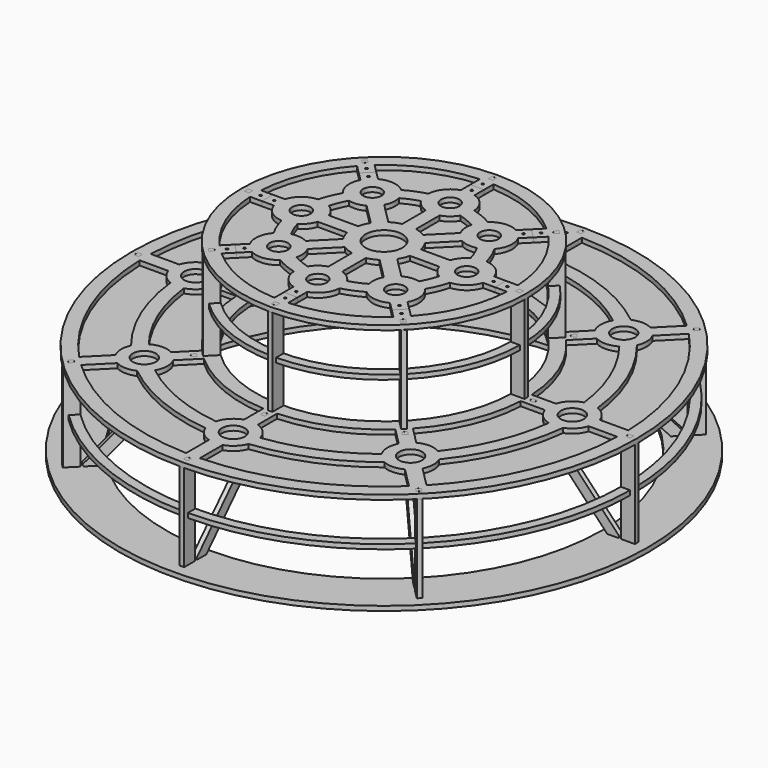
from build123d import *

# Parameters (mm, degrees)
F4_R      = 550
F4_R_2    = 25
F4_R_3    = 280
F5_DEPTH  = 10
F6_R      = 310
F6_R_2    = 2.5
F7_DEPTH  = 10
F8_R      = 575
F8_R_2    = 475
F9_DEPTH  = 10
F11_DEPTH = 5
F12_COUNT = 8
F13_R     = 520
F14_DEPTH = 10
F15_R     = 280
F16_DEPTH = 10
F17_COUNT = 8
F19_DEPTH = 1
F20_COUNT = 8
F6_R_3    = 20
F6_R_4    = 40
F21_DEPTH = 10
F23_DEPTH = 1
F24_COUNT = 4
F25_R     = 60
F26_DEPTH = 1


# Not quite as in the source:
# - the program builds the solid bodies; features that only make, move or delete a surface that nothing else refers to are left out


with BuildPart() as f5:
    # F4 (on Top) → F5 (new body)
    with BuildSketch(Plane.XY):
        Circle(F4_R)
        Polygon((-374.0594872477, -375.4737008101), (-371.3017708011, -378.2314172567), (-378.3728386129, -385.3024850685), (-381.1305550595, -382.5447686219), (-382.5447686219, -382.5447686219), (-382.5447686219, -381.1305550595), (-385.3024850685, -378.3728386129), (-378.2314172567, -371.3017708011), (-375.4737008101, -374.0594872477), (-374.0594872477, -374.0594872477), align=None, mode=Mode.SUBTRACT)
        with Locations((-289.9137802865, -289.9137802865)):
            Circle(F4_R_2, mode=Mode.SUBTRACT)
        with BuildLine():
            ThreePointArc((-46.8602222393, -427.4390243902), (-34.4319247471, -446.2552418033), (-15, -457.6969600708))
            Line((-15, -457.6969600708), (-15, -519.783608822))
            ThreePointArc((-15, -519.783608822), (-198.9953848298, -480.4173569059), (-356.9359128298, -378.1491162654))
            Line((-356.9359128298, -378.1491162654), (-313.0340224768, -334.2472259124))
            ThreePointArc((-313.0340224768, -334.2472259124), (-291.2030601412, -339.8971550971), (-269.1098517768, -335.3802136034))
            ThreePointArc((-269.1098517768, -335.3802136034), (-164.553875917, -397.2681989799), (-46.8602222393, -427.4390243902))
        make_face(mode=Mode.SUBTRACT)
        with BuildLine():
            Line((-15, -309.6368841078), (-15, -362.3030399292))
            ThreePointArc((-15, -362.3030399292), (-36.1104599854, -375.4162656782), (-48.3000733443, -397.0731707317))
            ThreePointArc((-48.3000733443, -397.0731707317), (-153.073372946, -369.5518130045), (-246.619822258, -314.9264410452))
            ThreePointArc((-246.619822258, -314.9264410452), (-239.9254361013, -290.9933383562), (-245.5803346606, -266.7935380962))
            Line((-245.5803346606, -266.7935380962), (-208.3397387403, -229.5529421759))
            ThreePointArc((-208.3397387403, -229.5529421759), (-118.6318640332, -286.4026550785), (-15, -309.6368841078))
        make_face(mode=Mode.SUBTRACT)
        with BuildLine():
            Line((-519.783608822, -15), (-457.6969600708, -15))
            ThreePointArc((-457.6969600708, -15), (-446.2552418033, -34.4319247471), (-427.4390243902, -46.8602222393))
            ThreePointArc((-427.4390243902, -46.8602222393), (-397.2681989799, -164.553875917), (-335.3802136034, -269.1098517768))
            ThreePointArc((-335.3802136034, -269.1098517768), (-339.8971550971, -291.2030601412), (-334.2472259124, -313.0340224768))
            Line((-334.2472259124, -313.0340224768), (-378.1491162654, -356.9359128298))
            ThreePointArc((-378.1491162654, -356.9359128298), (-480.4173569059, -198.9953848298), (-519.783608822, -15))
        make_face(mode=Mode.SUBTRACT)
        with BuildLine():
            ThreePointArc((-397.0731707317, -48.3000733443), (-375.4162656782, -36.1104599854), (-362.3030399292, -15))
            Line((-362.3030399292, -15), (-309.6368841078, -15))
            ThreePointArc((-309.6368841078, -15), (-286.4026550785, -118.6318640332), (-229.5529421759, -208.3397387403))
            Line((-229.5529421759, -208.3397387403), (-266.7935380962, -245.5803346606))
            ThreePointArc((-266.7935380962, -245.5803346606), (-290.9933383562, -239.9254361013), (-314.9264410452, -246.619822258))
            ThreePointArc((-314.9264410452, -246.619822258), (-369.5518130045, -153.073372946), (-397.0731707317, -48.3000733443))
        make_face(mode=Mode.SUBTRACT)
        Polygon((-236.8100610194, -229.8804145637), (-229.7389932075, -222.8093467519), (-226.9812767609, -225.5670631985), (-225.5670631985, -225.5670631985), (-225.5670631985, -226.9812767609), (-222.8093467519, -229.7389932075), (-229.8804145637, -236.8100610194), (-232.6381310104, -234.0523445727), (-234.0523445727, -234.0523445727), (-234.0523445727, -232.6381310104), align=None, mode=Mode.SUBTRACT)
        Polygon((-215.5968575838, -208.6672111282), (-208.5257897719, -201.5961433163), (-205.7680733253, -204.3538597629), (-204.3538597629, -204.3538597629), (-204.3538597629, -205.7680733253), (-201.5961433163, -208.5257897719), (-208.6672111282, -215.5968575838), (-211.4249275748, -212.8391411372), (-212.8391411372, -212.8391411372), (-212.8391411372, -211.4249275748), align=None, mode=Mode.SUBTRACT)
        Polygon((1, -530), (4.9, -530), (4.9, -540), (1, -540), (0, -541), (-1, -540), (-4.9, -540), (-4.9, -530), (-1, -530), (0, -529), align=None, mode=Mode.SUBTRACT)
        with BuildLine():
            ThreePointArc((356.9359128298, -378.1491162654), (198.9953848298, -480.4173569059), (15, -519.783608822))
            Line((15, -519.783608822), (15, -457.6969600708))
            ThreePointArc((15, -457.6969600708), (34.4319247471, -446.2552418033), (46.8602222393, -427.4390243902))
            ThreePointArc((46.8602222393, -427.4390243902), (164.553875917, -397.2681989799), (269.1098517768, -335.3802136034))
            ThreePointArc((269.1098517768, -335.3802136034), (291.2030601412, -339.8971550971), (313.0340224768, -334.2472259124))
            Line((313.0340224768, -334.2472259124), (356.9359128298, -378.1491162654))
        make_face(mode=Mode.SUBTRACT)
        with Locations((0, -410)):
            Circle(F4_R_2, mode=Mode.SUBTRACT)
        Polygon((-4.9, -330), (-4.9, -320), (-1, -320), (0, -319), (1, -320), (4.9, -320), (4.9, -330), (1, -330), (0, -331), (-1, -330), align=None, mode=Mode.SUBTRACT)
        Polygon((-4.9, -300), (-4.9, -290), (-1, -290), (0, -289), (1, -290), (4.9, -290), (4.9, -300), (1, -300), (0, -301), (-1, -300), align=None, mode=Mode.SUBTRACT)
        with BuildLine():
            ThreePointArc((246.619822258, -314.9264410452), (153.073372946, -369.5518130045), (48.3000733443, -397.0731707317))
            ThreePointArc((48.3000733443, -397.0731707317), (36.1104599854, -375.4162656782), (15, -362.3030399292))
            Line((15, -362.3030399292), (15, -309.6368841078))
            ThreePointArc((15, -309.6368841078), (118.6318640332, -286.4026550785), (208.3397387403, -229.5529421759))
            Line((208.3397387403, -229.5529421759), (245.5803346606, -266.7935380962))
            ThreePointArc((245.5803346606, -266.7935380962), (239.9254361013, -290.9933383562), (246.619822258, -314.9264410452))
        make_face(mode=Mode.SUBTRACT)
        Polygon((375.4737008101, -374.0594872477), (378.2314172567, -371.3017708011), (385.3024850685, -378.3728386129), (382.5447686219, -381.1305550595), (382.5447686219, -382.5447686219), (381.1305550595, -382.5447686219), (378.3728386129, -385.3024850685), (371.3017708011, -378.2314172567), (374.0594872477, -375.4737008101), (374.0594872477, -374.0594872477), align=None, mode=Mode.SUBTRACT)
        with Locations((289.9137802865, -289.9137802865)):
            Circle(F4_R_2, mode=Mode.SUBTRACT)
        Polygon((229.8804145637, -236.8100610194), (222.8093467519, -229.7389932075), (225.5670631985, -226.9812767609), (225.5670631985, -225.5670631985), (226.9812767609, -225.5670631985), (229.7389932075, -222.8093467519), (236.8100610194, -229.8804145637), (234.0523445727, -232.6381310104), (234.0523445727, -234.0523445727), (232.6381310104, -234.0523445727), align=None, mode=Mode.SUBTRACT)
        Polygon((208.6672111282, -215.5968575838), (201.5961433163, -208.5257897719), (204.3538597629, -205.7680733253), (204.3538597629, -204.3538597629), (205.7680733253, -204.3538597629), (208.5257897719, -201.5961433163), (215.5968575838, -208.6672111282), (212.8391411372, -211.4249275748), (212.8391411372, -212.8391411372), (211.4249275748, -212.8391411372), align=None, mode=Mode.SUBTRACT)
        with BuildLine():
            Line((378.1491162654, -356.9359128298), (334.2472259124, -313.0340224768))
            ThreePointArc((334.2472259124, -313.0340224768), (339.8971550971, -291.2030601412), (335.3802136034, -269.1098517768))
            ThreePointArc((335.3802136034, -269.1098517768), (397.2681989799, -164.553875917), (427.4390243902, -46.8602222393))
            ThreePointArc((427.4390243902, -46.8602222393), (446.2552418033, -34.4319247471), (457.6969600708, -15))
            Line((457.6969600708, -15), (519.783608822, -15))
            ThreePointArc((519.783608822, -15), (480.4173569059, -198.9953848298), (378.1491162654, -356.9359128298))
        make_face(mode=Mode.SUBTRACT)
        with BuildLine():
            ThreePointArc((314.9264410452, -246.619822258), (290.9933383562, -239.9254361013), (266.7935380962, -245.5803346606))
            Line((266.7935380962, -245.5803346606), (229.5529421759, -208.3397387403))
            ThreePointArc((229.5529421759, -208.3397387403), (286.4026550785, -118.6318640332), (309.6368841078, -15))
            Line((309.6368841078, -15), (362.3030399292, -15))
            ThreePointArc((362.3030399292, -15), (375.4162656782, -36.1104599854), (397.0731707317, -48.3000733443))
            ThreePointArc((397.0731707317, -48.3000733443), (369.5518130045, -153.073372946), (314.9264410452, -246.619822258))
        make_face(mode=Mode.SUBTRACT)
        Polygon((-530, -1), (-530, -4.9), (-540, -4.9), (-540, -1), (-541, 0), (-540, 1), (-540, 4.9), (-530, 4.9), (-530, 1), (-529, 0), align=None, mode=Mode.SUBTRACT)
        with Locations((-410, 0)):
            Circle(F4_R_2, mode=Mode.SUBTRACT)
        Polygon((-330, 4.9), (-320, 4.9), (-320, 1), (-319, 0), (-320, -1), (-320, -4.9), (-330, -4.9), (-330, -1), (-331, 0), (-330, 1), align=None, mode=Mode.SUBTRACT)
        Polygon((-300, 4.9), (-290, 4.9), (-290, 1), (-289, 0), (-290, -1), (-290, -4.9), (-300, -4.9), (-300, -1), (-301, 0), (-300, 1), align=None, mode=Mode.SUBTRACT)
        with BuildLine():
            ThreePointArc((-314.9264410452, 246.619822258), (-290.9933383562, 239.9254361013), (-266.7935380962, 245.5803346606))
            Line((-266.7935380962, 245.5803346606), (-229.5529421759, 208.3397387403))
            ThreePointArc((-229.5529421759, 208.3397387403), (-286.4026550785, 118.6318640332), (-309.6368841078, 15))
            Line((-309.6368841078, 15), (-362.3030399292, 15))
            ThreePointArc((-362.3030399292, 15), (-375.4162656782, 36.1104599854), (-397.0731707317, 48.3000733443))
            ThreePointArc((-397.0731707317, 48.3000733443), (-369.5518130045, 153.073372946), (-314.9264410452, 246.619822258))
        make_face(mode=Mode.SUBTRACT)
        with BuildLine():
            Line((-378.1491162654, 356.9359128298), (-334.2472259124, 313.0340224768))
            ThreePointArc((-334.2472259124, 313.0340224768), (-339.8971550971, 291.2030601412), (-335.3802136034, 269.1098517768))
            ThreePointArc((-335.3802136034, 269.1098517768), (-397.2681989799, 164.553875917), (-427.4390243902, 46.8602222393))
            ThreePointArc((-427.4390243902, 46.8602222393), (-446.2552418033, 34.4319247471), (-457.6969600708, 15))
            Line((-457.6969600708, 15), (-519.783608822, 15))
            ThreePointArc((-519.783608822, 15), (-480.4173569059, 198.9953848298), (-378.1491162654, 356.9359128298))
        make_face(mode=Mode.SUBTRACT)
        Polygon((-208.6672111282, 215.5968575838), (-201.5961433163, 208.5257897719), (-204.3538597629, 205.7680733253), (-204.3538597629, 204.3538597629), (-205.7680733253, 204.3538597629), (-208.5257897719, 201.5961433163), (-215.5968575838, 208.6672111282), (-212.8391411372, 211.4249275748), (-212.8391411372, 212.8391411372), (-211.4249275748, 212.8391411372), align=None, mode=Mode.SUBTRACT)
        Polygon((-229.8804145637, 236.8100610194), (-222.8093467519, 229.7389932075), (-225.5670631985, 226.9812767609), (-225.5670631985, 225.5670631985), (-226.9812767609, 225.5670631985), (-229.7389932075, 222.8093467519), (-236.8100610194, 229.8804145637), (-234.0523445727, 232.6381310104), (-234.0523445727, 234.0523445727), (-232.6381310104, 234.0523445727), align=None, mode=Mode.SUBTRACT)
        with Locations((-289.9137802865, 289.9137802865)):
            Circle(F4_R_2, mode=Mode.SUBTRACT)
        Polygon((-375.4737008101, 374.0594872477), (-378.2314172567, 371.3017708011), (-385.3024850685, 378.3728386129), (-382.5447686219, 381.1305550595), (-382.5447686219, 382.5447686219), (-381.1305550595, 382.5447686219), (-378.3728386129, 385.3024850685), (-371.3017708011, 378.2314172567), (-374.0594872477, 375.4737008101), (-374.0594872477, 374.0594872477), align=None, mode=Mode.SUBTRACT)
        with BuildLine():
            ThreePointArc((-48.3000733443, 397.0731707317), (-36.1104599854, 375.4162656782), (-15, 362.3030399292))
            Line((-15, 362.3030399292), (-15, 309.6368841078))
            ThreePointArc((-15, 309.6368841078), (-118.6318640332, 286.4026550785), (-208.3397387403, 229.5529421759))
            Line((-208.3397387403, 229.5529421759), (-245.5803346606, 266.7935380962))
            ThreePointArc((-245.5803346606, 266.7935380962), (-239.9254361013, 290.9933383562), (-246.619822258, 314.9264410452))
            ThreePointArc((-246.619822258, 314.9264410452), (-153.073372946, 369.5518130045), (-48.3000733443, 397.0731707317))
        make_face(mode=Mode.SUBTRACT)
        with BuildLine():
            Line((-15, 519.783608822), (-15, 457.6969600708))
            ThreePointArc((-15, 457.6969600708), (-34.4319247471, 446.2552418033), (-46.8602222393, 427.4390243902))
            ThreePointArc((-46.8602222393, 427.4390243902), (-164.553875917, 397.2681989799), (-269.1098517768, 335.3802136034))
            ThreePointArc((-269.1098517768, 335.3802136034), (-291.2030601412, 339.8971550971), (-313.0340224768, 334.2472259124))
            Line((-313.0340224768, 334.2472259124), (-356.9359128298, 378.1491162654))
            ThreePointArc((-356.9359128298, 378.1491162654), (-198.9953848298, 480.4173569059), (-15, 519.783608822))
        make_face(mode=Mode.SUBTRACT)
        Circle(F4_R_3, mode=Mode.SUBTRACT)
        Polygon((215.5968575838, 208.6672111282), (208.5257897719, 201.5961433163), (205.7680733253, 204.3538597629), (204.3538597629, 204.3538597629), (204.3538597629, 205.7680733253), (201.5961433163, 208.5257897719), (208.6672111282, 215.5968575838), (211.4249275748, 212.8391411372), (212.8391411372, 212.8391411372), (212.8391411372, 211.4249275748), align=None, mode=Mode.SUBTRACT)
        Polygon((236.8100610194, 229.8804145637), (229.7389932075, 222.8093467519), (226.9812767609, 225.5670631985), (225.5670631985, 225.5670631985), (225.5670631985, 226.9812767609), (222.8093467519, 229.7389932075), (229.8804145637, 236.8100610194), (232.6381310104, 234.0523445727), (234.0523445727, 234.0523445727), (234.0523445727, 232.6381310104), align=None, mode=Mode.SUBTRACT)
        Polygon((300, -4.9), (290, -4.9), (290, -1), (289, 0), (290, 1), (290, 4.9), (300, 4.9), (300, 1), (301, 0), (300, -1), align=None, mode=Mode.SUBTRACT)
        Polygon((330, -4.9), (320, -4.9), (320, -1), (319, 0), (320, 1), (320, 4.9), (330, 4.9), (330, 1), (331, 0), (330, -1), align=None, mode=Mode.SUBTRACT)
        with Locations((410, 0)):
            Circle(F4_R_2, mode=Mode.SUBTRACT)
        with BuildLine():
            ThreePointArc((397.0731707317, 48.3000733443), (375.4162656782, 36.1104599854), (362.3030399292, 15))
            Line((362.3030399292, 15), (309.6368841078, 15))
            ThreePointArc((309.6368841078, 15), (286.4026550785, 118.6318640332), (229.5529421759, 208.3397387403))
            Line((229.5529421759, 208.3397387403), (266.7935380962, 245.5803346606))
            ThreePointArc((266.7935380962, 245.5803346606), (290.9933383562, 239.9254361013), (314.9264410452, 246.619822258))
            ThreePointArc((314.9264410452, 246.619822258), (369.5518130045, 153.073372946), (397.0731707317, 48.3000733443))
        make_face(mode=Mode.SUBTRACT)
        Polygon((530, 1), (530, 4.9), (540, 4.9), (540, 1), (541, 0), (540, -1), (540, -4.9), (530, -4.9), (530, -1), (529, 0), align=None, mode=Mode.SUBTRACT)
        with BuildLine():
            Line((519.783608822, 15), (457.6969600708, 15))
            ThreePointArc((457.6969600708, 15), (446.2552418033, 34.4319247471), (427.4390243902, 46.8602222393))
            ThreePointArc((427.4390243902, 46.8602222393), (397.2681989799, 164.553875917), (335.3802136034, 269.1098517768))
            ThreePointArc((335.3802136034, 269.1098517768), (339.8971550971, 291.2030601412), (334.2472259124, 313.0340224768))
            Line((334.2472259124, 313.0340224768), (378.1491162654, 356.9359128298))
            ThreePointArc((378.1491162654, 356.9359128298), (480.4173569059, 198.9953848298), (519.783608822, 15))
        make_face(mode=Mode.SUBTRACT)
        Polygon((4.9, 300), (4.9, 290), (1, 290), (0, 289), (-1, 290), (-4.9, 290), (-4.9, 300), (-1, 300), (0, 301), (1, 300), align=None, mode=Mode.SUBTRACT)
        Polygon((4.9, 330), (4.9, 320), (1, 320), (0, 319), (-1, 320), (-4.9, 320), (-4.9, 330), (-1, 330), (0, 331), (1, 330), align=None, mode=Mode.SUBTRACT)
        with BuildLine():
            ThreePointArc((246.619822258, 314.9264410452), (239.9254361013, 290.9933383562), (245.5803346606, 266.7935380962))
            Line((245.5803346606, 266.7935380962), (208.3397387403, 229.5529421759))
            ThreePointArc((208.3397387403, 229.5529421759), (118.6318640332, 286.4026550785), (15, 309.6368841078))
            Line((15, 309.6368841078), (15, 362.3030399292))
            ThreePointArc((15, 362.3030399292), (36.1104599854, 375.4162656782), (48.3000733443, 397.0731707317))
            ThreePointArc((48.3000733443, 397.0731707317), (153.073372946, 369.5518130045), (246.619822258, 314.9264410452))
        make_face(mode=Mode.SUBTRACT)
        with Locations((0, 410)):
            Circle(F4_R_2, mode=Mode.SUBTRACT)
        Polygon((4.9, 540), (4.9, 530), (1, 530), (0, 529), (-1, 530), (-4.9, 530), (-4.9, 540), (-1, 540), (0, 541), (1, 540), align=None, mode=Mode.SUBTRACT)
        with BuildLine():
            Line((356.9359128298, 378.1491162654), (313.0340224768, 334.2472259124))
            ThreePointArc((313.0340224768, 334.2472259124), (291.2030601412, 339.8971550971), (269.1098517768, 335.3802136034))
            ThreePointArc((269.1098517768, 335.3802136034), (164.553875917, 397.2681989799), (46.8602222393, 427.4390243902))
            ThreePointArc((46.8602222393, 427.4390243902), (34.4319247471, 446.2552418033), (15, 457.6969600708))
            Line((15, 457.6969600708), (15, 519.783608822))
            ThreePointArc((15, 519.783608822), (198.9953848298, 480.4173569059), (356.9359128298, 378.1491162654))
        make_face(mode=Mode.SUBTRACT)
        with Locations((289.9137802865, 289.9137802865)):
            Circle(F4_R_2, mode=Mode.SUBTRACT)
        Polygon((374.0594872477, 375.4737008101), (371.3017708011, 378.2314172567), (378.3728386129, 385.3024850685), (381.1305550595, 382.5447686219), (382.5447686219, 382.5447686219), (382.5447686219, 381.1305550595), (385.3024850685, 378.3728386129), (378.2314172567, 371.3017708011), (375.4737008101, 374.0594872477), (374.0594872477, 374.0594872477), align=None, mode=Mode.SUBTRACT)
    extrude(amount=F5_DEPTH)


with BuildPart() as f7:
    # F6 (on offset) → F7 (new body)
    with BuildSketch(Plane.XY.offset(200)):
        Circle(F6_R)
        Polygon((-204.3538597629, -204.3538597629), (-204.3538597629, -205.7680733253), (-201.5961433163, -208.5257897719), (-208.6672111282, -215.5968575838), (-211.4249275748, -212.8391411372), (-212.8391411372, -212.8391411372), (-212.8391411372, -211.4249275748), (-215.5968575838, -208.6672111282), (-208.5257897719, -201.5961433163), (-205.7680733253, -204.3538597629), align=None, mode=Mode.SUBTRACT)
        with Locations((-189.9624285775, -189.9624285775)):
            Circle(F6_R_2, mode=Mode.SUBTRACT)
        Polygon((0, -289), (1, -290), (4.9, -290), (4.9, -300), (1, -300), (0, -301), (-1, -300), (-4.9, -300), (-4.9, -290), (-1, -290), align=None, mode=Mode.SUBTRACT)
        with Locations((0, -268.6474428356)):
            Circle(F6_R_2, mode=Mode.SUBTRACT)
        Polygon((204.3538597629, -204.3538597629), (205.7680733253, -204.3538597629), (208.5257897719, -201.5961433163), (215.5968575838, -208.6672111282), (212.8391411372, -211.4249275748), (212.8391411372, -212.8391411372), (211.4249275748, -212.8391411372), (208.6672111282, -215.5968575838), (201.5961433163, -208.5257897719), (204.3538597629, -205.7680733253), align=None, mode=Mode.SUBTRACT)
        with Locations((189.9624285775, -189.9624285775)):
            Circle(F6_R_2, mode=Mode.SUBTRACT)
        Polygon((-289, 0), (-290, -1), (-290, -4.9), (-300, -4.9), (-300, -1), (-301, 0), (-300, 1), (-300, 4.9), (-290, 4.9), (-290, 1), align=None, mode=Mode.SUBTRACT)
        with Locations((-268.6474428356, 0)):
            Circle(F6_R_2, mode=Mode.SUBTRACT)
        with Locations((-189.9624285775, 189.9624285775)):
            Circle(F6_R_2, mode=Mode.SUBTRACT)
        Polygon((-204.3538597629, 204.3538597629), (-205.7680733253, 204.3538597629), (-208.5257897719, 201.5961433163), (-215.5968575838, 208.6672111282), (-212.8391411372, 211.4249275748), (-212.8391411372, 212.8391411372), (-211.4249275748, 212.8391411372), (-208.6672111282, 215.5968575838), (-201.5961433163, 208.5257897719), (-204.3538597629, 205.7680733253), align=None, mode=Mode.SUBTRACT)
        with BuildLine():
            Line((15, -279.5979256003), (15, -253.6474428356))
            Line((15, -253.6474428356), (-15, -253.6474428356))
            Line((-15, -253.6474428356), (-15, -279.5979256003))
            ThreePointArc((-15, -279.5979256003), (-107.1513610622, -258.6862691032), (-187.0989874799, -208.3121909155))
            Line((-187.0989874799, -208.3121909155), (-168.7492251419, -189.9624285775))
            Line((-168.7492251419, -189.9624285775), (-189.9624285775, -168.7492251419))
            Line((-189.9624285775, -168.7492251419), (-208.3121909155, -187.0989874799))
            ThreePointArc((-208.3121909155, -187.0989874799), (-258.6862691032, -107.1513610622), (-279.5979256003, -15))
            Line((-279.5979256003, -15), (-253.6474428356, -15))
            Line((-253.6474428356, -15), (-253.6474428356, 15))
            Line((-253.6474428356, 15), (-279.5979256003, 15))
            ThreePointArc((-279.5979256003, 15), (-258.6862691032, 107.1513610622), (-208.3121909155, 187.0989874799))
            Line((-208.3121909155, 187.0989874799), (-189.9624285775, 168.7492251419))
            Line((-189.9624285775, 168.7492251419), (-168.7492251419, 189.9624285775))
            Line((-168.7492251419, 189.9624285775), (-187.0989874799, 208.3121909155))
            ThreePointArc((-187.0989874799, 208.3121909155), (-107.1513610622, 258.6862691032), (-15, 279.5979256003))
            Line((-15, 279.5979256003), (-15, 253.6474428356))
            Line((-15, 253.6474428356), (15, 253.6474428356))
            Line((15, 253.6474428356), (15, 279.5979256003))
            ThreePointArc((15, 279.5979256003), (107.1513610622, 258.6862691032), (187.0989874799, 208.3121909155))
            Line((187.0989874799, 208.3121909155), (168.7492251419, 189.9624285775))
            Line((168.7492251419, 189.9624285775), (189.9624285775, 168.7492251419))
            Line((189.9624285775, 168.7492251419), (208.3121909155, 187.0989874799))
            ThreePointArc((208.3121909155, 187.0989874799), (258.6862691032, 107.1513610622), (279.5979256003, 15))
            Line((279.5979256003, 15), (253.6474428356, 15))
            Line((253.6474428356, 15), (253.6474428356, -15))
            Line((253.6474428356, -15), (279.5979256003, -15))
            ThreePointArc((279.5979256003, -15), (258.6862691032, -107.1513610622), (208.3121909155, -187.0989874799))
            Line((208.3121909155, -187.0989874799), (189.9624285775, -168.7492251419))
            Line((189.9624285775, -168.7492251419), (168.7492251419, -189.9624285775))
            Line((168.7492251419, -189.9624285775), (187.0989874799, -208.3121909155))
            ThreePointArc((187.0989874799, -208.3121909155), (107.1513610622, -258.6862691032), (15, -279.5979256003))
        make_face(mode=Mode.SUBTRACT)
        with Locations((268.6474428356, 0)):
            Circle(F6_R_2, mode=Mode.SUBTRACT)
        Polygon((289, 0), (290, 1), (290, 4.9), (300, 4.9), (300, 1), (301, 0), (300, -1), (300, -4.9), (290, -4.9), (290, -1), align=None, mode=Mode.SUBTRACT)
        with Locations((0, 268.6474428356)):
            Circle(F6_R_2, mode=Mode.SUBTRACT)
        Polygon((-1, 290), (-4.9, 290), (-4.9, 300), (-1, 300), (0, 301), (1, 300), (4.9, 300), (4.9, 290), (1, 290), (0, 289), align=None, mode=Mode.SUBTRACT)
        with Locations((189.9624285775, 189.9624285775)):
            Circle(F6_R_2, mode=Mode.SUBTRACT)
        Polygon((204.3538597629, 204.3538597629), (204.3538597629, 205.7680733253), (201.5961433163, 208.5257897719), (208.6672111282, 215.5968575838), (211.4249275748, 212.8391411372), (212.8391411372, 212.8391411372), (212.8391411372, 211.4249275748), (215.5968575838, 208.6672111282), (208.5257897719, 201.5961433163), (205.7680733253, 204.3538597629), align=None, mode=Mode.SUBTRACT)
    extrude(amount=F7_DEPTH)


with BuildPart() as f9:
    # F8 (on offset) → F9 (new body)
    with BuildSketch(Plane.XY.offset(-200)):
        Circle(F8_R)
        Polygon((-374.0594872477, -375.4737008101), (-371.3017708011, -378.2314172567), (-378.3728386129, -385.3024850685), (-381.1305550595, -382.5447686219), (-382.5447686219, -382.5447686219), (-382.5447686219, -381.1305550595), (-385.3024850685, -378.3728386129), (-378.2314172567, -371.3017708011), (-375.4737008101, -374.0594872477), (-374.0594872477, -374.0594872477), align=None, mode=Mode.SUBTRACT)
        Polygon((-364.089281633, -357.1596351773), (-357.0182138211, -350.0885673655), (-354.2604973745, -352.8462838121), (-352.8462838121, -352.8462838121), (-352.8462838121, -354.2604973745), (-350.0885673655, -357.0182138211), (-357.1596351773, -364.089281633), (-359.917351624, -361.3315651863), (-361.3315651863, -361.3315651863), (-361.3315651863, -359.917351624), align=None, mode=Mode.SUBTRACT)
        Polygon((1, -530), (4.9, -530), (4.9, -540), (1, -540), (0, -541), (-1, -540), (-4.9, -540), (-4.9, -530), (-1, -530), (0, -529), align=None, mode=Mode.SUBTRACT)
        Polygon((-4.9, -510), (-4.9, -500), (-1, -500), (0, -499), (1, -500), (4.9, -500), (4.9, -510), (1, -510), (0, -511), (-1, -510), align=None, mode=Mode.SUBTRACT)
        Polygon((375.4737008101, -374.0594872477), (378.2314172567, -371.3017708011), (385.3024850685, -378.3728386129), (382.5447686219, -381.1305550595), (382.5447686219, -382.5447686219), (381.1305550595, -382.5447686219), (378.3728386129, -385.3024850685), (371.3017708011, -378.2314172567), (374.0594872477, -375.4737008101), (374.0594872477, -374.0594872477), align=None, mode=Mode.SUBTRACT)
        Polygon((357.1596351773, -364.089281633), (350.0885673655, -357.0182138211), (352.8462838121, -354.2604973745), (352.8462838121, -352.8462838121), (354.2604973745, -352.8462838121), (357.0182138211, -350.0885673655), (364.089281633, -357.1596351773), (361.3315651863, -359.917351624), (361.3315651863, -361.3315651863), (359.917351624, -361.3315651863), align=None, mode=Mode.SUBTRACT)
        Polygon((-530, -1), (-530, -4.9), (-540, -4.9), (-540, -1), (-541, 0), (-540, 1), (-540, 4.9), (-530, 4.9), (-530, 1), (-529, 0), align=None, mode=Mode.SUBTRACT)
        Polygon((-510, 4.9), (-500, 4.9), (-500, 1), (-499, 0), (-500, -1), (-500, -4.9), (-510, -4.9), (-510, -1), (-511, 0), (-510, 1), align=None, mode=Mode.SUBTRACT)
        Polygon((-357.1596351773, 364.089281633), (-350.0885673655, 357.0182138211), (-352.8462838121, 354.2604973745), (-352.8462838121, 352.8462838121), (-354.2604973745, 352.8462838121), (-357.0182138211, 350.0885673655), (-364.089281633, 357.1596351773), (-361.3315651863, 359.917351624), (-361.3315651863, 361.3315651863), (-359.917351624, 361.3315651863), align=None, mode=Mode.SUBTRACT)
        Polygon((-375.4737008101, 374.0594872477), (-378.2314172567, 371.3017708011), (-385.3024850685, 378.3728386129), (-382.5447686219, 381.1305550595), (-382.5447686219, 382.5447686219), (-381.1305550595, 382.5447686219), (-378.3728386129, 385.3024850685), (-371.3017708011, 378.2314172567), (-374.0594872477, 375.4737008101), (-374.0594872477, 374.0594872477), align=None, mode=Mode.SUBTRACT)
        Circle(F8_R_2, mode=Mode.SUBTRACT)
        Polygon((510, -4.9), (500, -4.9), (500, -1), (499, 0), (500, 1), (500, 4.9), (510, 4.9), (510, 1), (511, 0), (510, -1), align=None, mode=Mode.SUBTRACT)
        Polygon((530, 1), (530, 4.9), (540, 4.9), (540, 1), (541, 0), (540, -1), (540, -4.9), (530, -4.9), (530, -1), (529, 0), align=None, mode=Mode.SUBTRACT)
        Polygon((4.9, 510), (4.9, 500), (1, 500), (0, 499), (-1, 500), (-4.9, 500), (-4.9, 510), (-1, 510), (0, 511), (1, 510), align=None, mode=Mode.SUBTRACT)
        Polygon((4.9, 540), (4.9, 530), (1, 530), (0, 529), (-1, 530), (-4.9, 530), (-4.9, 540), (-1, 540), (0, 541), (1, 540), align=None, mode=Mode.SUBTRACT)
        Polygon((364.089281633, 357.1596351773), (357.0182138211, 350.0885673655), (354.2604973745, 352.8462838121), (352.8462838121, 352.8462838121), (352.8462838121, 354.2604973745), (350.0885673655, 357.0182138211), (357.1596351773, 364.089281633), (359.917351624, 361.3315651863), (361.3315651863, 361.3315651863), (361.3315651863, 359.917351624), align=None, mode=Mode.SUBTRACT)
        Polygon((374.0594872477, 375.4737008101), (371.3017708011, 378.2314172567), (378.3728386129, 385.3024850685), (381.1305550595, 382.5447686219), (382.5447686219, 382.5447686219), (382.5447686219, 381.1305550595), (385.3024850685, 378.3728386129), (378.2314172567, 371.3017708011), (375.4737008101, 374.0594872477), (374.0594872477, 374.0594872477), align=None, mode=Mode.SUBTRACT)
    extrude(amount=F9_DEPTH)


with BuildPart() as f11:
    # F10 (on Right) → F11 (new body, symmetric)
    with BuildSketch(Plane.YZ):
        Polygon((550, 0), (540, 0), (540, 10), (530, 10), (530, 0), (520, 0), (520, -90.1), (530, -90.1), (530, -99.9), (520, -99.9), (520, -190), (530, -190), (530, -200), (540, -200), (540, -190), (550, -190), align=None)
    extrude(amount=F11_DEPTH, both=True)


with BuildPart() as f11b:
    # F10 (on Right) → F11, piece 2 (new body, symmetric)
    with BuildSketch(Plane.YZ):
        Polygon((290, 10), (290, 0), (300, 0), (300, 10), (310, 10), (310, 200), (300, 200), (300, 210), (290, 210), (290, 200), (280, 200), (280, 109.9), (290, 109.9), (290, 100.1), (280, 100.1), (280, 10), align=None)
    extrude(amount=F11_DEPTH, both=True)


with BuildPart() as f11c:
    # F10 (on Right) → F11, piece 3 (new body, symmetric)
    with BuildSketch(Plane.YZ):
        with BuildLine():
            Line((510, -190), (513.0253940016, -190))
            ThreePointArc((513.0253940016, -190), (515.7812697092, -188.1853898449), (515.2032520533, -184.9367660563))
            Line((515.2032520533, -184.9367660563), (340, 0))
            Line((340, 0), (330, 0))
            Line((330, 0), (330, 10))
            Line((330, 10), (320, 10))
            Line((320, 10), (320, 0))
            Line((320, 0), (310, 0))
            Line((310, 0), (490, -190))
            Line((490, -190), (500, -190))
            Line((500, -190), (500, -200))
            Line((500, -200), (510, -200))
            Line((510, -200), (510, -190))
        make_face()
    extrude(amount=F11_DEPTH, both=True)


with BuildPart() as f12_1:
    # F12: instance of F11
    add(f11.part.rotate(Axis((0, 0, 200), (0, 0, 1)), 1 * 360 / F12_COUNT))


with BuildPart() as f12_2:
    # F12: instance of F11
    add(f11.part.rotate(Axis((0, 0, 200), (0, 0, 1)), 2 * 360 / F12_COUNT))


with BuildPart() as f12_3:
    # F12: instance of F11
    add(f11.part.rotate(Axis((0, 0, 200), (0, 0, 1)), 3 * 360 / F12_COUNT))


with BuildPart() as f12_4:
    # F12: instance of F11
    add(f11.part.rotate(Axis((0, 0, 200), (0, 0, 1)), 4 * 360 / F12_COUNT))


with BuildPart() as f12_5:
    # F12: instance of F11
    add(f11.part.rotate(Axis((0, 0, 200), (0, 0, 1)), 5 * 360 / F12_COUNT))


with BuildPart() as f12_6:
    # F12: instance of F11
    add(f11.part.rotate(Axis((0, 0, 200), (0, 0, 1)), 6 * 360 / F12_COUNT))


with BuildPart() as f12_7:
    # F12: instance of F11
    add(f11.part.rotate(Axis((0, 0, 200), (0, 0, 1)), 7 * 360 / F12_COUNT))


with BuildPart() as f12_8:
    # F12: instance of F11b
    add(f11b.part.rotate(Axis((0, 0, 200), (0, 0, 1)), 1 * 360 / F12_COUNT))


with BuildPart() as f12_9:
    # F12: instance of F11b
    add(f11b.part.rotate(Axis((0, 0, 200), (0, 0, 1)), 2 * 360 / F12_COUNT))


with BuildPart() as f12_10:
    # F12: instance of F11b
    add(f11b.part.rotate(Axis((0, 0, 200), (0, 0, 1)), 3 * 360 / F12_COUNT))


with BuildPart() as f12_11:
    # F12: instance of F11b
    add(f11b.part.rotate(Axis((0, 0, 200), (0, 0, 1)), 4 * 360 / F12_COUNT))


with BuildPart() as f12_12:
    # F12: instance of F11b
    add(f11b.part.rotate(Axis((0, 0, 200), (0, 0, 1)), 5 * 360 / F12_COUNT))


with BuildPart() as f12_13:
    # F12: instance of F11b
    add(f11b.part.rotate(Axis((0, 0, 200), (0, 0, 1)), 6 * 360 / F12_COUNT))


with BuildPart() as f12_14:
    # F12: instance of F11b
    add(f11b.part.rotate(Axis((0, 0, 200), (0, 0, 1)), 7 * 360 / F12_COUNT))


with BuildPart() as f14:
    # F13 (on offset) → F14 (new body)
    with BuildSketch(Plane.XY.offset(-100)):
        with BuildLine():
            Line((-530, -5), (-539.9768513557, -5))
            ThreePointArc((-539.9768513557, -5), (-498.8949475561, -206.6490534771), (-385.3568271833, -378.2857593714))
            Line((-385.3568271833, -378.2857593714), (-378.3021279348, -371.2310601229))
            Line((-378.3021279348, -371.2310601229), (-371.2310601229, -378.3021279348))
            Line((-371.2310601229, -378.3021279348), (-378.2857593714, -385.3568271833))
            ThreePointArc((-378.2857593714, -385.3568271833), (-206.6490534771, -498.8949475561), (-5, -539.9768513557))
            Line((-5, -539.9768513557), (-5, -530))
            Line((-5, -530), (5, -530))
            Line((5, -530), (5, -539.9768513557))
            ThreePointArc((5, -539.9768513557), (206.6490534771, -498.8949475561), (378.2857593714, -385.3568271833))
            Line((378.2857593714, -385.3568271833), (371.2310601229, -378.3021279348))
            Line((371.2310601229, -378.3021279348), (378.3021279348, -371.2310601229))
            Line((378.3021279348, -371.2310601229), (385.3568271833, -378.2857593714))
            ThreePointArc((385.3568271833, -378.2857593714), (498.8949475561, -206.6490534771), (539.9768513557, -5))
            Line((539.9768513557, -5), (530, -5))
            Line((530, -5), (530, 5))
            Line((530, 5), (539.9768513557, 5))
            ThreePointArc((539.9768513557, 5), (498.8949475561, 206.6490534771), (385.3568271833, 378.2857593714))
            Line((385.3568271833, 378.2857593714), (378.3021279348, 371.2310601229))
            Line((378.3021279348, 371.2310601229), (371.2310601229, 378.3021279348))
            Line((371.2310601229, 378.3021279348), (378.2857593714, 385.3568271833))
            ThreePointArc((378.2857593714, 385.3568271833), (206.6490534771, 498.8949475561), (5, 539.9768513557))
            Line((5, 539.9768513557), (5, 530))
            Line((5, 530), (-5, 530))
            Line((-5, 530), (-5, 539.9768513557))
            ThreePointArc((-5, 539.9768513557), (-206.6490534771, 498.8949475561), (-378.2857593714, 385.3568271833))
            Line((-378.2857593714, 385.3568271833), (-371.2310601229, 378.3021279348))
            Line((-371.2310601229, 378.3021279348), (-378.3021279348, 371.2310601229))
            Line((-378.3021279348, 371.2310601229), (-385.3568271833, 378.2857593714))
            ThreePointArc((-385.3568271833, 378.2857593714), (-498.8949475561, 206.6490534771), (-539.9768513557, 5))
            Line((-539.9768513557, 5), (-530, 5))
            Line((-530, 5), (-530, -5))
        make_face()
        Circle(F13_R, mode=Mode.SUBTRACT)
    extrude(amount=F14_DEPTH)


with BuildPart() as f16:
    # F15 (on offset) → F16 (new body)
    with BuildSketch(Plane.XY.offset(100)):
        with BuildLine():
            Line((-290, -5), (-299.9583304394, -5))
            ThreePointArc((-299.9583304394, -5), (-277.1638597534, -114.8050297095), (-215.638103433, -208.5670356212))
            Line((-215.638103433, -208.5670356212), (-208.59650045, -201.5254326382))
            Line((-208.59650045, -201.5254326382), (-201.5254326382, -208.59650045))
            Line((-201.5254326382, -208.59650045), (-208.5670356212, -215.638103433))
            ThreePointArc((-208.5670356212, -215.638103433), (-114.8050297095, -277.1638597534), (-5, -299.9583304394))
            Line((-5, -299.9583304394), (-5, -290))
            Line((-5, -290), (5, -290))
            Line((5, -290), (5, -299.9583304394))
            ThreePointArc((5, -299.9583304394), (114.8050297095, -277.1638597534), (208.5670356212, -215.638103433))
            Line((208.5670356212, -215.638103433), (201.5254326382, -208.59650045))
            Line((201.5254326382, -208.59650045), (208.59650045, -201.5254326382))
            Line((208.59650045, -201.5254326382), (215.638103433, -208.5670356212))
            ThreePointArc((215.638103433, -208.5670356212), (277.1638597534, -114.8050297095), (299.9583304394, -5))
            Line((299.9583304394, -5), (290, -5))
            Line((290, -5), (290, 5))
            Line((290, 5), (299.9583304394, 5))
            ThreePointArc((299.9583304394, 5), (277.1638597534, 114.8050297095), (215.638103433, 208.5670356212))
            Line((215.638103433, 208.5670356212), (208.59650045, 201.5254326382))
            Line((208.59650045, 201.5254326382), (201.5254326382, 208.59650045))
            Line((201.5254326382, 208.59650045), (208.5670356212, 215.638103433))
            ThreePointArc((208.5670356212, 215.638103433), (114.8050297095, 277.1638597534), (5, 299.9583304394))
            Line((5, 299.9583304394), (5, 290))
            Line((5, 290), (-5, 290))
            Line((-5, 290), (-5, 299.9583304394))
            ThreePointArc((-5, 299.9583304394), (-114.8050297095, 277.1638597534), (-208.5670356212, 215.638103433))
            Line((-208.5670356212, 215.638103433), (-201.5254326382, 208.59650045))
            Line((-201.5254326382, 208.59650045), (-208.59650045, 201.5254326382))
            Line((-208.59650045, 201.5254326382), (-215.638103433, 208.5670356212))
            ThreePointArc((-215.638103433, 208.5670356212), (-277.1638597534, 114.8050297095), (-299.9583304394, 5))
            Line((-299.9583304394, 5), (-290, 5))
            Line((-290, 5), (-290, -5))
        make_face()
        Circle(F15_R, mode=Mode.SUBTRACT)
    extrude(amount=F16_DEPTH)


with BuildPart() as f17_1:
    # F17: instance of F11c
    add(f11c.part.rotate(Axis((0, 0, 0), (0, 0, 1)), 1 * 360 / F17_COUNT))


with BuildPart() as f17_2:
    # F17: instance of F11c
    add(f11c.part.rotate(Axis((0, 0, 0), (0, 0, 1)), 2 * 360 / F17_COUNT))


with BuildPart() as f17_3:
    # F17: instance of F11c
    add(f11c.part.rotate(Axis((0, 0, 0), (0, 0, 1)), 3 * 360 / F17_COUNT))


with BuildPart() as f17_4:
    # F17: instance of F11c
    add(f11c.part.rotate(Axis((0, 0, 0), (0, 0, 1)), 4 * 360 / F17_COUNT))


with BuildPart() as f17_5:
    # F17: instance of F11c
    add(f11c.part.rotate(Axis((0, 0, 0), (0, 0, 1)), 5 * 360 / F17_COUNT))


with BuildPart() as f17_6:
    # F17: instance of F11c
    add(f11c.part.rotate(Axis((0, 0, 0), (0, 0, 1)), 6 * 360 / F17_COUNT))


with BuildPart() as f17_7:
    # F17: instance of F11c
    add(f11c.part.rotate(Axis((0, 0, 0), (0, 0, 1)), 7 * 360 / F17_COUNT))


with BuildPart() as f19:
    # F18 (on face) → F19 (new body)
    with BuildSketch(Plane(origin=(0, 0, 0), x_dir=(1, 0, 0), z_dir=(0, 0, -1))):
        with BuildLine():
            ThreePointArc((368.3698207303, 378.2693156669), (202.0568522888, 487.808393166), (7, 527.9535964457))
            Line((7, 527.9535964457), (7, 451.4125584817))
            ThreePointArc((7, 451.4125584817), (42, 410), (7, 368.5874415183))
            Line((7, 368.5874415183), (7, 301.9188632729))
            ThreePointArc((7, 301.9188632729), (115.5703965743, 279.0116188184), (208.5391281201, 218.4386230567))
            Line((208.5391281201, 218.4386230567), (255.6809318895, 265.5804268261))
            ThreePointArc((255.6809318895, 265.5804268261), (319.6122650963, 260.2152954766), (314.2471337469, 324.1466286835))
            Line((314.2471337469, 324.1466286835), (368.3698207303, 378.2693156669))
        make_face()
    extrude(amount=F19_DEPTH)


with BuildPart() as f20_1:
    # F20: instance of F19
    add(f19.part.rotate(Axis((0, 0, 0), (0, 0, 1)), 1 * 360 / F20_COUNT))


with BuildPart() as f20_2:
    # F20: instance of F19
    add(f19.part.rotate(Axis((0, 0, 0), (0, 0, 1)), 2 * 360 / F20_COUNT))


with BuildPart() as f20_3:
    # F20: instance of F19
    add(f19.part.rotate(Axis((0, 0, 0), (0, 0, 1)), 3 * 360 / F20_COUNT))


with BuildPart() as f20_4:
    # F20: instance of F19
    add(f19.part.rotate(Axis((0, 0, 0), (0, 0, 1)), 4 * 360 / F20_COUNT))


with BuildPart() as f20_5:
    # F20: instance of F19
    add(f19.part.rotate(Axis((0, 0, 0), (0, 0, 1)), 5 * 360 / F20_COUNT))


with BuildPart() as f20_6:
    # F20: instance of F19
    add(f19.part.rotate(Axis((0, 0, 0), (0, 0, 1)), 6 * 360 / F20_COUNT))


with BuildPart() as f20_7:
    # F20: instance of F19
    add(f19.part.rotate(Axis((0, 0, 0), (0, 0, 1)), 7 * 360 / F20_COUNT))


with BuildPart() as f21:
    # F6 (on offset) → F21 (new body)
    with BuildSketch(Plane.XY.offset(200)):
        with BuildLine():
            ThreePointArc((15, -227.6969600708), (39.3023002536, -210.9084000682), (49.888765157, -183.3333333333))
            ThreePointArc((49.888765157, -183.3333333333), (72.7098521494, -175.5371111771), (94.35955907, -164.9129273651))
            ThreePointArc((94.35955907, -164.9129273651), (121.3438368718, -176.925682923), (150.3994628039, -171.6126662395))
            Line((150.3994628039, -171.6126662395), (168.7492251419, -189.9624285775))
            Line((168.7492251419, -189.9624285775), (189.9624285775, -168.7492251419))
            Line((189.9624285775, -168.7492251419), (171.6126662395, -150.3994628039))
            ThreePointArc((171.6126662395, -150.3994628039), (176.925682923, -121.3438368718), (164.9129273651, -94.35955907))
            ThreePointArc((164.9129273651, -94.35955907), (175.5371111771, -72.7098521494), (183.3333333333, -49.888765157))
            ThreePointArc((183.3333333333, -49.888765157), (210.9084000682, -39.3023002536), (227.6969600708, -15))
            Line((227.6969600708, -15), (253.6474428356, -15))
            Line((253.6474428356, -15), (253.6474428356, 15))
            Line((253.6474428356, 15), (227.6969600708, 15))
            ThreePointArc((227.6969600708, 15), (210.9084000682, 39.3023002536), (183.3333333333, 49.888765157))
            ThreePointArc((183.3333333333, 49.888765157), (175.5371111771, 72.7098521494), (164.9129273651, 94.35955907))
            ThreePointArc((164.9129273651, 94.35955907), (176.925682923, 121.3438368718), (171.6126662395, 150.3994628039))
            Line((171.6126662395, 150.3994628039), (189.9624285775, 168.7492251419))
            Line((189.9624285775, 168.7492251419), (168.7492251419, 189.9624285775))
            Line((168.7492251419, 189.9624285775), (150.3994628039, 171.6126662395))
            ThreePointArc((150.3994628039, 171.6126662395), (121.3438368718, 176.925682923), (94.35955907, 164.9129273651))
            ThreePointArc((94.35955907, 164.9129273651), (72.7098521494, 175.5371111771), (49.888765157, 183.3333333333))
            ThreePointArc((49.888765157, 183.3333333333), (39.3023002536, 210.9084000682), (15, 227.6969600708))
            Line((15, 227.6969600708), (15, 253.6474428356))
            Line((15, 253.6474428356), (-15, 253.6474428356))
            Line((-15, 253.6474428356), (-15, 227.6969600708))
            ThreePointArc((-15, 227.6969600708), (-39.3023002536, 210.9084000682), (-49.888765157, 183.3333333333))
            ThreePointArc((-49.888765157, 183.3333333333), (-72.7098521494, 175.5371111771), (-94.35955907, 164.9129273651))
            ThreePointArc((-94.35955907, 164.9129273651), (-121.3438368718, 176.925682923), (-150.3994628039, 171.6126662395))
            Line((-150.3994628039, 171.6126662395), (-168.7492251419, 189.9624285775))
            Line((-168.7492251419, 189.9624285775), (-189.9624285775, 168.7492251419))
            Line((-189.9624285775, 168.7492251419), (-171.6126662395, 150.3994628039))
            ThreePointArc((-171.6126662395, 150.3994628039), (-176.925682923, 121.3438368718), (-164.9129273651, 94.35955907))
            ThreePointArc((-164.9129273651, 94.35955907), (-175.5371111771, 72.7098521494), (-183.3333333333, 49.888765157))
            ThreePointArc((-183.3333333333, 49.888765157), (-210.9084000682, 39.3023002536), (-227.6969600708, 15))
            Line((-227.6969600708, 15), (-253.6474428356, 15))
            Line((-253.6474428356, 15), (-253.6474428356, -15))
            Line((-253.6474428356, -15), (-227.6969600708, -15))
            ThreePointArc((-227.6969600708, -15), (-210.9084000682, -39.3023002536), (-183.3333333333, -49.888765157))
            ThreePointArc((-183.3333333333, -49.888765157), (-175.5371111771, -72.7098521494), (-164.9129273651, -94.35955907))
            ThreePointArc((-164.9129273651, -94.35955907), (-176.925682923, -121.3438368718), (-171.6126662395, -150.3994628039))
            Line((-171.6126662395, -150.3994628039), (-189.9624285775, -168.7492251419))
            Line((-189.9624285775, -168.7492251419), (-168.7492251419, -189.9624285775))
            Line((-168.7492251419, -189.9624285775), (-150.3994628039, -171.6126662395))
            ThreePointArc((-150.3994628039, -171.6126662395), (-121.3438368718, -176.925682923), (-94.35955907, -164.9129273651))
            ThreePointArc((-94.35955907, -164.9129273651), (-72.7098521494, -175.5371111771), (-49.888765157, -183.3333333333))
            ThreePointArc((-49.888765157, -183.3333333333), (-39.3023002536, -210.9084000682), (-15, -227.6969600708))
            Line((-15, -227.6969600708), (-15, -253.6474428356))
            Line((-15, -253.6474428356), (15, -253.6474428356))
            Line((15, -253.6474428356), (15, -227.6969600708))
        make_face()
        with Locations((-168.7492251419, -168.7492251419)):
            Circle(F6_R_2, mode=Mode.SUBTRACT)
        with Locations((-127.2792206136, -127.2792206136)):
            Circle(F6_R_3, mode=Mode.SUBTRACT)
        with BuildLine():
            Line((-15, -68.3739716559), (-15, -132.3030399292))
            ThreePointArc((-15, -132.3030399292), (-30.9028195191, -140.6933116916), (-42.8093317968, -154.1666666667))
            ThreePointArc((-42.8093317968, -154.1666666667), (-61.2293491784, -147.8207252018), (-78.7415266213, -139.2830642445))
            ThreePointArc((-78.7415266213, -139.2830642445), (-77.633601525, -121.3367880044), (-82.9457749877, -104.1589784233))
            Line((-82.9457749877, -104.1589784233), (-37.7410972967, -58.9543007323))
            ThreePointArc((-37.7410972967, -58.9543007323), (-26.7878402656, -64.6715672758), (-15, -68.3739716559))
        make_face(mode=Mode.SUBTRACT)
        with BuildLine():
            Line((-132.3030399292, -15), (-68.3739716559, -15))
            ThreePointArc((-68.3739716559, -15), (-64.6715672758, -26.7878402656), (-58.9543007323, -37.7410972967))
            Line((-58.9543007323, -37.7410972967), (-104.1589784233, -82.9457749877))
            ThreePointArc((-104.1589784233, -82.9457749877), (-121.3367880044, -77.633601525), (-139.2830642445, -78.7415266213))
            ThreePointArc((-139.2830642445, -78.7415266213), (-147.8207252018, -61.2293491784), (-154.1666666667, -42.8093317968))
            ThreePointArc((-154.1666666667, -42.8093317968), (-140.6933116916, -30.9028195191), (-132.3030399292, -15))
        make_face(mode=Mode.SUBTRACT)
        with Locations((0, -238.6474428356)):
            Circle(F6_R_2, mode=Mode.SUBTRACT)
        with Locations((0, -180)):
            Circle(F6_R_3, mode=Mode.SUBTRACT)
        with Locations((168.7492251419, -168.7492251419)):
            Circle(F6_R_2, mode=Mode.SUBTRACT)
        with BuildLine():
            ThreePointArc((78.7415266213, -139.2830642445), (61.2293491784, -147.8207252018), (42.8093317968, -154.1666666667))
            ThreePointArc((42.8093317968, -154.1666666667), (30.9028195191, -140.6933116916), (15, -132.3030399292))
            Line((15, -132.3030399292), (15, -68.3739716559))
            ThreePointArc((15, -68.3739716559), (26.7878402656, -64.6715672758), (37.7410972967, -58.9543007323))
            Line((37.7410972967, -58.9543007323), (82.9457749877, -104.1589784233))
            ThreePointArc((82.9457749877, -104.1589784233), (77.633601525, -121.3367880044), (78.7415266213, -139.2830642445))
        make_face(mode=Mode.SUBTRACT)
        with Locations((127.2792206136, -127.2792206136)):
            Circle(F6_R_3, mode=Mode.SUBTRACT)
        with BuildLine():
            Line((104.1589784233, -82.9457749877), (58.9543007323, -37.7410972967))
            ThreePointArc((58.9543007323, -37.7410972967), (64.6715672758, -26.7878402656), (68.3739716559, -15))
            Line((68.3739716559, -15), (132.3030399292, -15))
            ThreePointArc((132.3030399292, -15), (140.6933116916, -30.9028195191), (154.1666666667, -42.8093317968))
            ThreePointArc((154.1666666667, -42.8093317968), (147.8207252018, -61.2293491784), (139.2830642445, -78.7415266213))
            ThreePointArc((139.2830642445, -78.7415266213), (121.3367880044, -77.633601525), (104.1589784233, -82.9457749877))
        make_face(mode=Mode.SUBTRACT)
        with Locations((-238.6474428356, 0)):
            Circle(F6_R_2, mode=Mode.SUBTRACT)
        with Locations((-180, 0)):
            Circle(F6_R_3, mode=Mode.SUBTRACT)
        with BuildLine():
            Line((-104.1589784233, 82.9457749877), (-58.9543007323, 37.7410972967))
            ThreePointArc((-58.9543007323, 37.7410972967), (-64.6715672758, 26.7878402656), (-68.3739716559, 15))
            Line((-68.3739716559, 15), (-132.3030399292, 15))
            ThreePointArc((-132.3030399292, 15), (-140.6933116916, 30.9028195191), (-154.1666666667, 42.8093317968))
            ThreePointArc((-154.1666666667, 42.8093317968), (-147.8207252018, 61.2293491784), (-139.2830642445, 78.7415266213))
            ThreePointArc((-139.2830642445, 78.7415266213), (-121.3367880044, 77.633601525), (-104.1589784233, 82.9457749877))
        make_face(mode=Mode.SUBTRACT)
        with Locations((-127.2792206136, 127.2792206136)):
            Circle(F6_R_3, mode=Mode.SUBTRACT)
        with BuildLine():
            Line((-15, 132.3030399292), (-15, 68.3739716559))
            ThreePointArc((-15, 68.3739716559), (-26.7878402656, 64.6715672758), (-37.7410972967, 58.9543007323))
            Line((-37.7410972967, 58.9543007323), (-82.9457749877, 104.1589784233))
            ThreePointArc((-82.9457749877, 104.1589784233), (-77.633601525, 121.3367880044), (-78.7415266213, 139.2830642445))
            ThreePointArc((-78.7415266213, 139.2830642445), (-61.2293491784, 147.8207252018), (-42.8093317968, 154.1666666667))
            ThreePointArc((-42.8093317968, 154.1666666667), (-30.9028195191, 140.6933116916), (-15, 132.3030399292))
        make_face(mode=Mode.SUBTRACT)
        with Locations((-168.7492251419, 168.7492251419)):
            Circle(F6_R_2, mode=Mode.SUBTRACT)
        Circle(F6_R_4, mode=Mode.SUBTRACT)
        with BuildLine():
            Line((132.3030399292, 15), (68.3739716559, 15))
            ThreePointArc((68.3739716559, 15), (64.6715672758, 26.7878402656), (58.9543007323, 37.7410972967))
            Line((58.9543007323, 37.7410972967), (104.1589784233, 82.9457749877))
            ThreePointArc((104.1589784233, 82.9457749877), (121.3367880044, 77.633601525), (139.2830642445, 78.7415266213))
            ThreePointArc((139.2830642445, 78.7415266213), (147.8207252018, 61.2293491784), (154.1666666667, 42.8093317968))
            ThreePointArc((154.1666666667, 42.8093317968), (140.6933116916, 30.9028195191), (132.3030399292, 15))
        make_face(mode=Mode.SUBTRACT)
        with BuildLine():
            Line((82.9457749877, 104.1589784233), (37.7410972967, 58.9543007323))
            ThreePointArc((37.7410972967, 58.9543007323), (26.7878402656, 64.6715672758), (15, 68.3739716559))
            Line((15, 68.3739716559), (15, 132.3030399292))
            ThreePointArc((15, 132.3030399292), (30.9028195191, 140.6933116916), (42.8093317968, 154.1666666667))
            ThreePointArc((42.8093317968, 154.1666666667), (61.2293491784, 147.8207252018), (78.7415266213, 139.2830642445))
            ThreePointArc((78.7415266213, 139.2830642445), (77.633601525, 121.3367880044), (82.9457749877, 104.1589784233))
        make_face(mode=Mode.SUBTRACT)
        with Locations((127.2792206136, 127.2792206136)):
            Circle(F6_R_3, mode=Mode.SUBTRACT)
        with Locations((180, 0)):
            Circle(F6_R_3, mode=Mode.SUBTRACT)
        with Locations((238.6474428356, 0)):
            Circle(F6_R_2, mode=Mode.SUBTRACT)
        with Locations((0, 180)):
            Circle(F6_R_3, mode=Mode.SUBTRACT)
        with Locations((0, 238.6474428356)):
            Circle(F6_R_2, mode=Mode.SUBTRACT)
        with Locations((168.7492251419, 168.7492251419)):
            Circle(F6_R_2, mode=Mode.SUBTRACT)
    extrude(amount=F21_DEPTH)


with BuildPart() as f23:
    # F22 (on face) → F23 (new body)
    with BuildSketch(Plane(origin=(0, 0, 200), x_dir=(1, 0, 0), z_dir=(0, 0, -1))):
        with BuildLine():
            ThreePointArc((287.9149179879, 7), (203.6467529817, 203.6467529817), (7, 287.9149179879))
            Line((7, 287.9149179879), (7, 221.4125584817))
            ThreePointArc((7, 221.4125584817), (42, 180), (7, 138.5874415183))
            Line((7, 138.5874415183), (7, 61.603571325))
            ThreePointArc((7, 61.603571325), (48.5100504976, 38.6105555609), (61.603571325, -7))
            Line((61.603571325, -7), (138.5874415183, -7))
            ThreePointArc((138.5874415183, -7), (187, -41.4125584817), (221.4125584817, 7))
            Line((221.4125584817, 7), (287.9149179879, 7))
        make_face()
    extrude(amount=F23_DEPTH)


with BuildPart() as f24_1:
    # F24: instance of F23
    add(f23.part.rotate(Axis((0, 0, 200), (0, 0, 1)), 1 * 360 / F24_COUNT))


with BuildPart() as f24_2:
    # F24: instance of F23
    add(f23.part.rotate(Axis((0, 0, 200), (0, 0, 1)), 2 * 360 / F24_COUNT))


with BuildPart() as f24_3:
    # F24: instance of F23
    add(f23.part.rotate(Axis((0, 0, 200), (0, 0, 1)), 3 * 360 / F24_COUNT))


with BuildPart() as f26:
    # F25 (on face) → F26 (new body)
    with BuildSketch(Plane(origin=(0, 0, 200), x_dir=(1, 0, 0), z_dir=(0, 0, -1))):
        Circle(F25_R)
    extrude(amount=F26_DEPTH)


solid = Compound([f5.part, f7.part, f9.part, f11.part, f11b.part, f11c.part, f12_1.part, f12_2.part, f12_3.part, f12_4.part, f12_5.part, f12_6.part, f12_7.part, f12_8.part, f12_9.part, f12_10.part, f12_11.part, f12_12.part, f12_13.part, f12_14.part, f14.part, f16.part, f17_1.part, f17_2.part, f17_3.part, f17_4.part, f17_5.part, f17_6.part, f17_7.part, f19.part, f20_1.part, f20_2.part, f20_3.part, f20_4.part, f20_5.part, f20_6.part, f20_7.part, f21.part, f23.part, f24_1.part, f24_2.part, f24_3.part, f26.part])
